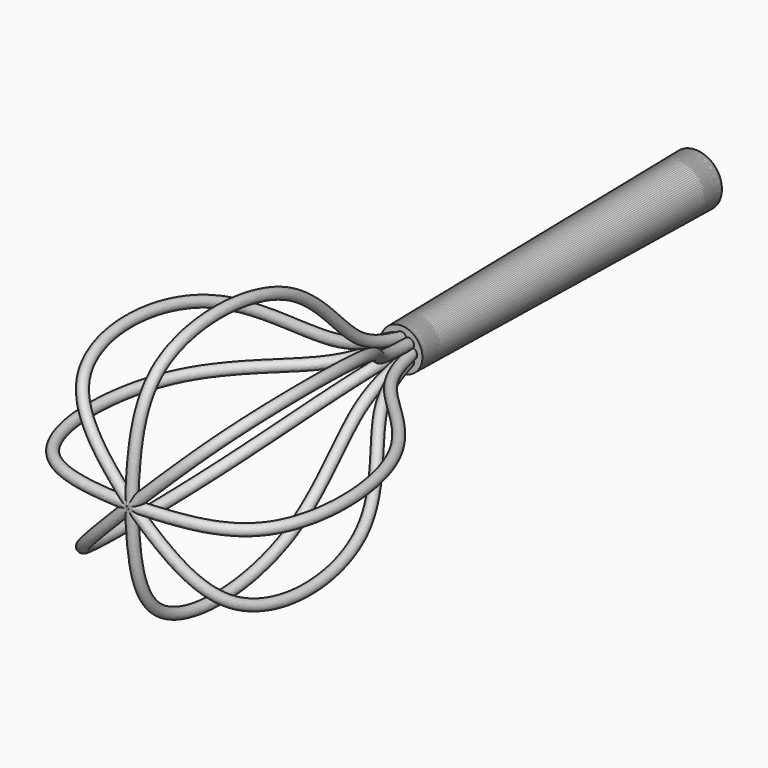
from build123d import *

# Parameters (mm, degrees)
F0_R     = 12.7
F2_R     = 10.16
F4_R     = 2.54
F8_COUNT = 8


with BuildPart() as f3:
    # F0 (on Front) → F3 section 0
    with BuildSketch(Plane.XZ):
        Circle(F0_R)
    # F2 (on offset) → F3 section 1
    with BuildSketch(Plane.XZ.offset(177.8)):
        Circle(F2_R)
    loft()

    # F6: sweep along a path in F5
    with BuildLine(Plane.YZ) as f6_path:
        add(Plane.YZ * Edge.make_bspline(
            [(-177.8, 5.0828022463), (-186.7715960901, 7.3008696134), (-208.3553090567, 12.6370582818), (-240.5956435574, 62.7631469867), (-336.9192687022, 65.0778785745), (-339.6309543694, 20.4402346711), (-340.8726751804, 0)],
            knots=[0, 0, 0, 0, 0.1847510921, 0.4444710286, 0.7456151009, 1, 1, 1, 1], degree=3))
    # F4 (on face) → F6 (sweep)
    with BuildSketch(Plane.XZ.offset(177.8)):
        with Locations((0, 5.0828022463)):
            Circle(F4_R)
    sweep(path=f6_path.line)


with BuildPart() as f8_1:
    # F8: instance of F3
    add(f3.part.rotate(Axis((0, -130.2067488432, 0), (0, -1, 0)), 1 * 360 / F8_COUNT))


with BuildPart() as f8_2:
    # F8: instance of F3
    add(f3.part.rotate(Axis((0, -130.2067488432, 0), (0, -1, 0)), 2 * 360 / F8_COUNT))


with BuildPart() as f8_3:
    # F8: instance of F3
    add(f3.part.rotate(Axis((0, -130.2067488432, 0), (0, -1, 0)), 3 * 360 / F8_COUNT))


with BuildPart() as f8_4:
    # F8: instance of F3
    add(f3.part.rotate(Axis((0, -130.2067488432, 0), (0, -1, 0)), 4 * 360 / F8_COUNT))


with BuildPart() as f8_5:
    # F8: instance of F3
    add(f3.part.rotate(Axis((0, -130.2067488432, 0), (0, -1, 0)), 5 * 360 / F8_COUNT))


with BuildPart() as f8_6:
    # F8: instance of F3
    add(f3.part.rotate(Axis((0, -130.2067488432, 0), (0, -1, 0)), 6 * 360 / F8_COUNT))


with BuildPart() as f8_7:
    # F8: instance of F3
    add(f3.part.rotate(Axis((0, -130.2067488432, 0), (0, -1, 0)), 7 * 360 / F8_COUNT))


solid = Compound([f3.part, f8_1.part, f8_2.part, f8_3.part, f8_4.part, f8_5.part, f8_6.part, f8_7.part])
